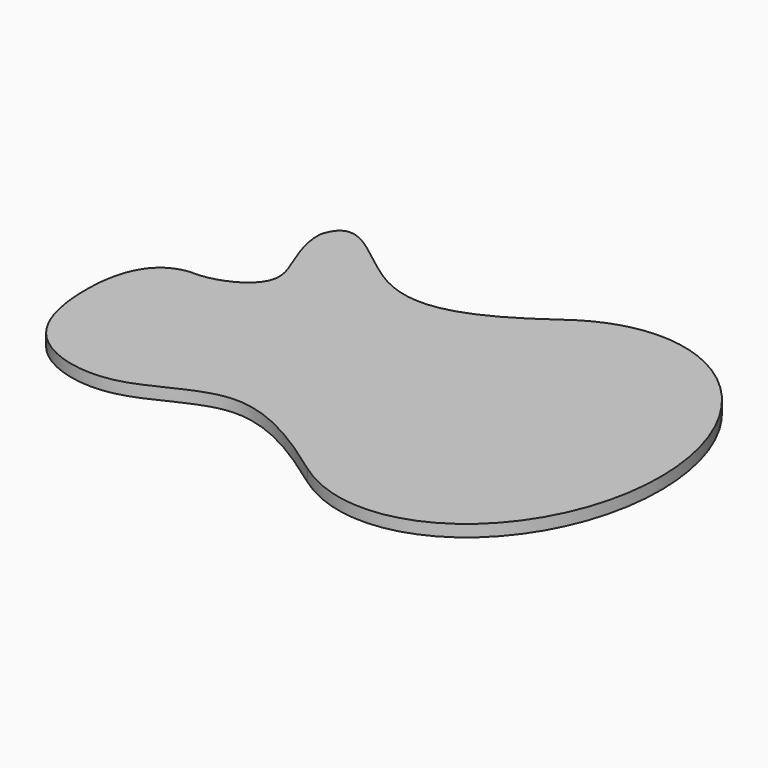
from build123d import *

# Parameters (mm, degrees)
F1_DEPTH = 8


with BuildPart() as f1:
    # F0 (on Top) → F1 (new body)
    with BuildSketch(Plane.XY):
        with BuildLine():
            add(Edge.make_bspline(
                [(71.8108263604, -123.8465007597), (47.7003894889, -106.5138372126), (-7.1023466925, -67.7010548051), (-65.7469849132, -118.3312863438), (-132.354363187, -102.6557773389), (-144.8947489305, -66.4196911039), (-145.8762223824, -43.2833050614)],
                knots=[0, 0, 0, 0, 0.2870393338, 0.537090623, 0.7679648384, 1, 1, 1, 1], degree=3))
            add(Edge.make_bspline(
                [(71.8108263604, -123.8465007597), (221.9776217834, -231.7995748847), (221.9776217834, -15.5333050614), (221.9776217834, 200.732964762), (71.8108263604, 92.7798906369)],
                knots=[2.6189550017, 2.6189550017, 2.6189550017, 4.7123889804, 4.7123889804, 6.805822959, 6.805822959, 6.805822959], degree=2, weights=[1, 0.500416121, 1, 0.500416121, 1]))
            add(Edge.make_bspline(
                [(71.8108263604, 92.7798906369), (32.8723456502, 64.787494425), (-21.3027110814, 39.7461116108), (-81.2909620858, 117.5857035406), (-89.3733802445, 87.9502004857)],
                knots=[0, 0, 0, 0, 0.5650436037, 1, 1, 1, 1], degree=3))
            add(Edge.make_bspline(
                [(-89.3733802445, 87.9502004857), (-90.0934642677, 65.0933156509), (-57.859468156, 30.7219399995), (-99.6368888097, 11.3485391097), (-115.4622438558, 12.2166949386)],
                knots=[0, 0, 0, 0, 0.5319080677, 1, 1, 1, 1], degree=3))
            add(Edge.make_bspline(
                [(-115.4622438558, 12.2166949386), (-140.0598439582, 10.2222937221), (-147.0534109131, -15.5333050614), (-145.8762223824, -43.2833050614)],
                knots=[0, 0, 0, 0, 63.2871242025, 63.2871242025, 63.2871242025, 63.2871242025], degree=3))
        make_face()
        with BuildLine():
            add(Edge.make_bspline(
                [(-81.4262804577, 86.6857544237), (-81.4396250825, 86.2899525598), (-81.470808458, 84.4412359429), (-81.2371444329, 80.3732443352), (-79.8996394846, 74.5622458053), (-77.7739796116, 68.1004270996), (-75.1889101521, 61.6875748493), (-72.6363769897, 55.6379909817), (-70.5528201855, 50.214885946), (-69.2861786808, 45.7296293686), (-68.4936431345, 42.0817923462), (-68.1698884875, 39.0929607397), (-68.1533657536, 36.6406286998), (-68.2570236145, 34.6616403838), (-68.4737574041, 33.0838263382), (-68.7291671623, 31.8176398216), (-68.9833432916, 30.7603115144), (-69.2894446793, 29.7143907955), (-69.7010474162, 28.4802252803), (-70.3057430461, 26.9847588782), (-71.2217272744, 25.180071771), (-72.5057098447, 22.996441344), (-74.3801649871, 20.4643430051), (-77.1315209855, 17.5971889856), (-80.926011463, 14.2754710831), (-86.2805957531, 10.7907129486), (-92.9455256658, 7.7447804381), (-100.4062506896, 5.4313702506), (-107.2615908321, 4.1555616419), (-112.3230611682, 4.0215517798), (-114.7617028131, 4.1430335828), (-115.474366372, 4.1953856873)],
                knots=[1.0136586156, 1.0136586156, 1.0136586156, 1.0136586156, 2.2016566853, 6.5591151943, 13.1979354067, 20.0157728224, 26.9584341349, 33.9306395999, 39.7192874549, 44.3702545919, 47.8991910145, 50.9066466506, 53.369227998, 55.2496065506, 56.847005284, 58.1419089398, 59.1235009163, 60.1084144557, 61.4103265818, 63.0253022922, 64.9424016715, 67.4766146145, 70.6177002822, 74.3676557464, 79.3769786716, 85.7174213089, 93.458168517, 101.2822181349, 109.1089736004, 114.2877981192, 116.4315649936, 116.4315649936, 116.4315649936, 116.4315649936], degree=3))
            add(Edge.make_bspline(
                [(72.8103885596, 83.6341241639), (71.1240314332, 82.4184487748), (65.3211296449, 78.2511465746), (54.3822197437, 70.6703789871), (40.5843185437, 63.3369671226), (27.1044447549, 57.4124251533), (15.6068408566, 53.964757392), (5.3548644478, 52.6151050201), (-2.8177310259, 52.7103819348), (-9.6197612713, 53.363557714), (-15.7305931996, 54.5996218363), (-21.4732164128, 56.31783797), (-26.4693776174, 58.366991406), (-30.2671336771, 60.2223905595), (-33.0718752326, 61.7320886712), (-35.2053892899, 62.9792168629), (-37.3369452365, 64.2673631998), (-39.7615979324, 65.8275673276), (-42.7778265582, 67.9000785118), (-46.5332653234, 70.5849117526), (-51.0723794993, 74.0383260586), (-56.0224963865, 77.9290754702), (-61.0223620617, 81.8442891195), (-65.7064727807, 85.3502794992), (-69.7594173643, 88.139955985), (-72.9865417062, 89.9814861225), (-75.2118467434, 90.9665662194), (-76.6921868128, 91.4830508838), (-77.6909621365, 91.7169743843), (-78.3366022017, 91.7578979554), (-78.6767300882, 91.7470455298), (-78.7973913091, 91.6896137336), (-78.92482237, 91.6464959623), (-79.1937851984, 91.3963059685), (-79.6818827943, 90.8264140362), (-80.3159105632, 89.7215409417), (-80.9369473577, 88.2993059967), (-81.2772034526, 87.2085598356), (-81.4244737614, 86.692097536), (-81.4262804577, 86.6857544237)],
                knots=[4.5292135135, 4.5292135135, 4.5292135135, 4.5292135135, 10.7658667308, 25.9500108525, 44.4238690912, 57.5330245622, 70.0845168555, 80.2898579631, 88.4222588801, 94.5557392843, 100.7652771107, 107.0947805516, 112.5088206902, 116.9457400715, 119.7701488038, 122.0625237383, 124.3588459686, 127.2414612751, 130.7107153436, 135.3368293125, 141.0894801607, 147.8190536406, 154.2256313175, 160.1398760262, 165.3706560057, 168.9759235223, 171.2693919986, 172.6578901032, 173.6814113013, 174.3231622883, 174.6136969662, 174.6729508701, 174.7225491593, 175.0159838788, 175.7405361192, 176.9913533667, 178.804034025, 180.3944536329, 180.4142282457, 180.4142282457, 180.4142282457, 180.4142282457], degree=3))
            add(Edge.make_bspline(
                [(72.8103885596, 83.6341241639), (72.7317618823, 83.5699644288), (70.9554937476, 82.1155753179), (67.9804833382, 79.4874285922), (64.1756082657, 75.8169878196), (61.2913248025, 72.7059934358), (59.0477069928, 70.0999739159), (57.2057633336, 67.8641883266), (55.4110672881, 65.56108087), (53.3041635287, 62.7354150513), (50.7805389552, 59.0881516023), (47.799656336, 54.2715974255), (44.2346711733, 47.9787195772), (40.2649118491, 39.7160179142), (36.5713092348, 29.8478370438), (33.5979528322, 19.5919068023), (31.7307948184, 10.2422116085), (30.6840668384, 2.616404127), (30.0568619889, -3.4886245577), (29.7723767309, -8.3519176651), (29.6597520537, -12.2635801323), (29.6233030189, -15.5333050614), (29.6597520537, -18.8030299904), (29.7723767309, -22.7146924576), (30.0568619889, -27.577985565), (30.6840668384, -33.6830142497), (31.7307948184, -41.3088217312), (33.5979528322, -50.658516925), (36.5713092348, -60.9144471666), (40.2649118491, -70.7826280369), (44.2346711733, -79.0453296999), (47.799656336, -85.3382075482), (50.7805389552, -90.154761725), (53.3041635287, -93.802025174), (55.4110672881, -96.6276909927), (57.2057633336, -98.9307984493), (59.0477069928, -101.1665840385), (61.2913248025, -103.7726035588), (64.1756082657, -106.8835979408), (67.9804833382, -110.5540387225), (71.0158561736, -113.2355100421), (72.8564442573, -114.7385263129), (72.9977731483, -114.8532271387)],
                knots=[55.4205486123, 55.4205486123, 55.4205486123, 55.4205486123, 55.7249011544, 62.305727762, 67.3238088056, 71.5787205888, 75.0272954709, 77.639141403, 80.2683237903, 83.7858930003, 88.2122067644, 93.5690542346, 100.7734603115, 109.9018351329, 121.0375002369, 132.3448319226, 141.8998601689, 149.6118137579, 155.4302714584, 160.3068693677, 164.2227012809, 167.1693695094, 170.1160377378, 174.0318696511, 178.9084675603, 184.7269252608, 192.4388788498, 201.9939070962, 213.3012387819, 224.4369038858, 233.5652787073, 240.7696847841, 246.1265322543, 250.5528460185, 254.0704152284, 256.6995976157, 259.3114435479, 262.76001843, 267.0149302132, 272.0330112567, 278.6138378644, 279.1597054143, 279.1597054143, 279.1597054143, 279.1597054143], degree=3))
            add(Edge.make_bspline(
                [(72.9977731483, -114.8532271387), (72.4056865049, -114.4263580428), (69.0464376439, -111.9992044047), (61.9105909681, -106.8036530478), (52.1940425374, -100.414675291), (42.2398177459, -94.2326232769), (33.0541391905, -89.1692992659), (24.2243642947, -84.9672989241), (16.2683766941, -82.0032951161), (9.8318873834, -80.2250290854), (4.463169856, -79.0636225581), (-0.1263073791, -78.4111921814), (-4.1937519975, -78.1649162686), (-7.7060356334, -78.20526396), (-11.1805991563, -78.3727848605), (-15.105690951, -78.8390498977), (-19.429069468, -79.71105596), (-23.8718019577, -80.9066029792), (-28.6468717479, -82.5067792162), (-34.2116599911, -84.6249302975), (-40.8658871469, -87.6398905134), (-47.690965404, -91.0045722285), (-53.9322172369, -94.031755035), (-58.8517886529, -96.1862154004), (-62.8636912858, -97.8099974599), (-66.2287548358, -99.0112055596), (-69.174479199, -99.8882996602), (-71.7101157046, -100.5041409348), (-74.2391141536, -101.045908585), (-77.1889902033, -101.5211815466), (-80.5636006609, -101.8380782168), (-84.1498166568, -101.9648655282), (-88.1283425241, -101.8479910003), (-92.8713789939, -101.4573804411), (-98.6786686768, -100.4434986326), (-104.6143126843, -98.6675537845), (-109.8122869472, -96.3889800651), (-113.6612373405, -94.2262164294), (-116.6721363111, -92.2928397642), (-119.445929644, -90.1897015323), (-122.5417365002, -87.5069010735), (-126.0053703089, -83.7372187502), (-129.3000799141, -78.8269050802), (-132.2206720517, -72.9997696435), (-134.760402105, -65.6917432119), (-136.8528161109, -57.6024378465), (-137.649866694, -49.6245863229), (-137.8414579174, -44.9060106494), (-137.8834109174, -42.9442403412)],
                knots=[4.2858061399, 4.2858061399, 4.2858061399, 4.2858061399, 6.4754935696, 16.7181495974, 30.7634466026, 41.3498570357, 51.8646712584, 62.2141493558, 70.6575747754, 77.2977144197, 82.2304258348, 87.1280777725, 91.1888826436, 94.4417008039, 97.6615312024, 101.6210664508, 106.2864985952, 110.880412158, 115.4145221345, 121.3894131446, 128.7352744437, 137.3194350468, 144.219174491, 149.5422059689, 153.4280250406, 157.2015215054, 160.2566826573, 162.6437031168, 165.0279610064, 168.0144585226, 171.6015387383, 175.1893400883, 178.772742133, 183.5366693447, 189.4556710281, 196.4255332119, 202.067982696, 206.4456583082, 209.6586104968, 212.7949457303, 216.8805616296, 221.934808933, 228.1024059287, 234.5573044306, 241.4332004742, 251.2825478576, 259.5402388761, 265.4359196068, 265.4359196068, 265.4359196068, 265.4359196068], degree=3))
            add(Edge.make_bspline(
                [(-115.474366372, 4.1953856873), (-115.654699102, 4.1804409153), (-116.5836359717, 4.0950636678), (-118.5079216061, 3.8241612148), (-121.094735833, 3.0439396902), (-123.6838235375, 1.8597581111), (-125.9853889989, 0.3481336416), (-128.0619952594, -1.4951736511), (-129.9535460087, -3.6932073495), (-131.8514714309, -6.5803447016), (-133.9637161202, -10.6180046655), (-136.0486166412, -16.5975276115), (-137.4710871628, -24.3656867863), (-138.1549681717, -32.3234699475), (-138.079170547, -38.6118374717), (-137.939859331, -41.8534729549), (-137.8834109174, -42.9442403412)],
                knots=[0.6605528161, 0.6605528161, 0.6605528161, 0.6605528161, 1.2032828879, 3.4574616871, 6.4791602651, 9.2718264149, 11.9726703823, 14.7076610425, 17.5762809491, 20.6455316793, 25.0544251668, 31.2157003257, 39.5600454386, 48.6812593878, 55.1351477368, 58.4131045259, 58.4131045259, 58.4131045259, 58.4131045259], degree=3))
        make_face(mode=Mode.SUBTRACT)
        with BuildLine():
            add(Edge.make_bspline(
                [(72.8103885596, 83.6341241639), (71.1240314332, 82.4184487748), (65.3211296449, 78.2511465746), (54.3822197437, 70.6703789871), (40.5843185437, 63.3369671226), (27.1044447549, 57.4124251533), (15.6068408566, 53.964757392), (5.3548644478, 52.6151050201), (-2.8177310259, 52.7103819348), (-9.6197612713, 53.363557714), (-15.7305931996, 54.5996218363), (-21.4732164128, 56.31783797), (-26.4693776174, 58.366991406), (-30.2671336771, 60.2223905595), (-33.0718752326, 61.7320886712), (-35.2053892899, 62.9792168629), (-37.3369452365, 64.2673631998), (-39.7615979324, 65.8275673276), (-42.7778265582, 67.9000785118), (-46.5332653234, 70.5849117526), (-51.0723794993, 74.0383260586), (-56.0224963865, 77.9290754702), (-61.0223620617, 81.8442891195), (-65.7064727807, 85.3502794992), (-69.7594173643, 88.139955985), (-72.9865417062, 89.9814861225), (-75.2118467434, 90.9665662194), (-76.6921868128, 91.4830508838), (-77.6909621365, 91.7169743843), (-78.3366022017, 91.7578979554), (-78.6767300882, 91.7470455298), (-78.7973913091, 91.6896137336), (-78.92482237, 91.6464959623), (-79.1937851984, 91.3963059685), (-79.6818827943, 90.8264140362), (-80.3159105632, 89.7215409417), (-80.9369473577, 88.2993059967), (-81.2772034526, 87.2085598356), (-81.4244737614, 86.692097536), (-81.4262804577, 86.6857544237)],
                knots=[4.5292135135, 4.5292135135, 4.5292135135, 4.5292135135, 10.7658667308, 25.9500108525, 44.4238690912, 57.5330245622, 70.0845168555, 80.2898579631, 88.4222588801, 94.5557392843, 100.7652771107, 107.0947805516, 112.5088206902, 116.9457400715, 119.7701488038, 122.0625237383, 124.3588459686, 127.2414612751, 130.7107153436, 135.3368293125, 141.0894801607, 147.8190536406, 154.2256313175, 160.1398760262, 165.3706560057, 168.9759235223, 171.2693919986, 172.6578901032, 173.6814113013, 174.3231622883, 174.6136969662, 174.6729508701, 174.7225491593, 175.0159838788, 175.7405361192, 176.9913533667, 178.804034025, 180.3944536329, 180.4142282457, 180.4142282457, 180.4142282457, 180.4142282457], degree=3))
            add(Edge.make_bspline(
                [(-81.4262804577, 86.6857544237), (-81.4396250825, 86.2899525598), (-81.470808458, 84.4412359429), (-81.2371444329, 80.3732443352), (-79.8996394846, 74.5622458053), (-77.7739796116, 68.1004270996), (-75.1889101521, 61.6875748493), (-72.6363769897, 55.6379909817), (-70.5528201855, 50.214885946), (-69.2861786808, 45.7296293686), (-68.4936431345, 42.0817923462), (-68.1698884875, 39.0929607397), (-68.1533657536, 36.6406286998), (-68.2570236145, 34.6616403838), (-68.4737574041, 33.0838263382), (-68.7291671623, 31.8176398216), (-68.9833432916, 30.7603115144), (-69.2894446793, 29.7143907955), (-69.7010474162, 28.4802252803), (-70.3057430461, 26.9847588782), (-71.2217272744, 25.180071771), (-72.5057098447, 22.996441344), (-74.3801649871, 20.4643430051), (-77.1315209855, 17.5971889856), (-80.926011463, 14.2754710831), (-86.2805957531, 10.7907129486), (-92.9455256658, 7.7447804381), (-100.4062506896, 5.4313702506), (-107.2615908321, 4.1555616419), (-112.3230611682, 4.0215517798), (-114.7617028131, 4.1430335828), (-115.474366372, 4.1953856873)],
                knots=[1.0136586156, 1.0136586156, 1.0136586156, 1.0136586156, 2.2016566853, 6.5591151943, 13.1979354067, 20.0157728224, 26.9584341349, 33.9306395999, 39.7192874549, 44.3702545919, 47.8991910145, 50.9066466506, 53.369227998, 55.2496065506, 56.847005284, 58.1419089398, 59.1235009163, 60.1084144557, 61.4103265818, 63.0253022922, 64.9424016715, 67.4766146145, 70.6177002822, 74.3676557464, 79.3769786716, 85.7174213089, 93.458168517, 101.2822181349, 109.1089736004, 114.2877981192, 116.4315649936, 116.4315649936, 116.4315649936, 116.4315649936], degree=3))
            add(Edge.make_bspline(
                [(-115.474366372, 4.1953856873), (-115.654699102, 4.1804409153), (-116.5836359717, 4.0950636678), (-118.5079216061, 3.8241612148), (-121.094735833, 3.0439396902), (-123.6838235375, 1.8597581111), (-125.9853889989, 0.3481336416), (-128.0619952594, -1.4951736511), (-129.9535460087, -3.6932073495), (-131.8514714309, -6.5803447016), (-133.9637161202, -10.6180046655), (-136.0486166412, -16.5975276115), (-137.4710871628, -24.3656867863), (-138.1549681717, -32.3234699475), (-138.079170547, -38.6118374717), (-137.939859331, -41.8534729549), (-137.8834109174, -42.9442403412)],
                knots=[0.6605528161, 0.6605528161, 0.6605528161, 0.6605528161, 1.2032828879, 3.4574616871, 6.4791602651, 9.2718264149, 11.9726703823, 14.7076610425, 17.5762809491, 20.6455316793, 25.0544251668, 31.2157003257, 39.5600454386, 48.6812593878, 55.1351477368, 58.4131045259, 58.4131045259, 58.4131045259, 58.4131045259], degree=3))
            add(Edge.make_bspline(
                [(72.9977731483, -114.8532271387), (72.4056865049, -114.4263580428), (69.0464376439, -111.9992044047), (61.9105909681, -106.8036530478), (52.1940425374, -100.414675291), (42.2398177459, -94.2326232769), (33.0541391905, -89.1692992659), (24.2243642947, -84.9672989241), (16.2683766941, -82.0032951161), (9.8318873834, -80.2250290854), (4.463169856, -79.0636225581), (-0.1263073791, -78.4111921814), (-4.1937519975, -78.1649162686), (-7.7060356334, -78.20526396), (-11.1805991563, -78.3727848605), (-15.105690951, -78.8390498977), (-19.429069468, -79.71105596), (-23.8718019577, -80.9066029792), (-28.6468717479, -82.5067792162), (-34.2116599911, -84.6249302975), (-40.8658871469, -87.6398905134), (-47.690965404, -91.0045722285), (-53.9322172369, -94.031755035), (-58.8517886529, -96.1862154004), (-62.8636912858, -97.8099974599), (-66.2287548358, -99.0112055596), (-69.174479199, -99.8882996602), (-71.7101157046, -100.5041409348), (-74.2391141536, -101.045908585), (-77.1889902033, -101.5211815466), (-80.5636006609, -101.8380782168), (-84.1498166568, -101.9648655282), (-88.1283425241, -101.8479910003), (-92.8713789939, -101.4573804411), (-98.6786686768, -100.4434986326), (-104.6143126843, -98.6675537845), (-109.8122869472, -96.3889800651), (-113.6612373405, -94.2262164294), (-116.6721363111, -92.2928397642), (-119.445929644, -90.1897015323), (-122.5417365002, -87.5069010735), (-126.0053703089, -83.7372187502), (-129.3000799141, -78.8269050802), (-132.2206720517, -72.9997696435), (-134.760402105, -65.6917432119), (-136.8528161109, -57.6024378465), (-137.649866694, -49.6245863229), (-137.8414579174, -44.9060106494), (-137.8834109174, -42.9442403412)],
                knots=[4.2858061399, 4.2858061399, 4.2858061399, 4.2858061399, 6.4754935696, 16.7181495974, 30.7634466026, 41.3498570357, 51.8646712584, 62.2141493558, 70.6575747754, 77.2977144197, 82.2304258348, 87.1280777725, 91.1888826436, 94.4417008039, 97.6615312024, 101.6210664508, 106.2864985952, 110.880412158, 115.4145221345, 121.3894131446, 128.7352744437, 137.3194350468, 144.219174491, 149.5422059689, 153.4280250406, 157.2015215054, 160.2566826573, 162.6437031168, 165.0279610064, 168.0144585226, 171.6015387383, 175.1893400883, 178.772742133, 183.5366693447, 189.4556710281, 196.4255332119, 202.067982696, 206.4456583082, 209.6586104968, 212.7949457303, 216.8805616296, 221.934808933, 228.1024059287, 234.5573044306, 241.4332004742, 251.2825478576, 259.5402388761, 265.4359196068, 265.4359196068, 265.4359196068, 265.4359196068], degree=3))
            add(Edge.make_bspline(
                [(72.8103885596, 83.6341241639), (72.7317618823, 83.5699644288), (70.9554937476, 82.1155753179), (67.9804833382, 79.4874285922), (64.1756082657, 75.8169878196), (61.2913248025, 72.7059934358), (59.0477069928, 70.0999739159), (57.2057633336, 67.8641883266), (55.4110672881, 65.56108087), (53.3041635287, 62.7354150513), (50.7805389552, 59.0881516023), (47.799656336, 54.2715974255), (44.2346711733, 47.9787195772), (40.2649118491, 39.7160179142), (36.5713092348, 29.8478370438), (33.5979528322, 19.5919068023), (31.7307948184, 10.2422116085), (30.6840668384, 2.616404127), (30.0568619889, -3.4886245577), (29.7723767309, -8.3519176651), (29.6597520537, -12.2635801323), (29.6233030189, -15.5333050614), (29.6597520537, -18.8030299904), (29.7723767309, -22.7146924576), (30.0568619889, -27.577985565), (30.6840668384, -33.6830142497), (31.7307948184, -41.3088217312), (33.5979528322, -50.658516925), (36.5713092348, -60.9144471666), (40.2649118491, -70.7826280369), (44.2346711733, -79.0453296999), (47.799656336, -85.3382075482), (50.7805389552, -90.154761725), (53.3041635287, -93.802025174), (55.4110672881, -96.6276909927), (57.2057633336, -98.9307984493), (59.0477069928, -101.1665840385), (61.2913248025, -103.7726035588), (64.1756082657, -106.8835979408), (67.9804833382, -110.5540387225), (71.0158561736, -113.2355100421), (72.8564442573, -114.7385263129), (72.9977731483, -114.8532271387)],
                knots=[55.4205486123, 55.4205486123, 55.4205486123, 55.4205486123, 55.7249011544, 62.305727762, 67.3238088056, 71.5787205888, 75.0272954709, 77.639141403, 80.2683237903, 83.7858930003, 88.2122067644, 93.5690542346, 100.7734603115, 109.9018351329, 121.0375002369, 132.3448319226, 141.8998601689, 149.6118137579, 155.4302714584, 160.3068693677, 164.2227012809, 167.1693695094, 170.1160377378, 174.0318696511, 178.9084675603, 184.7269252608, 192.4388788498, 201.9939070962, 213.3012387819, 224.4369038858, 233.5652787073, 240.7696847841, 246.1265322543, 250.5528460185, 254.0704152284, 256.6995976157, 259.3114435479, 262.76001843, 267.0149302132, 272.0330112567, 278.6138378644, 279.1597054143, 279.1597054143, 279.1597054143, 279.1597054143], degree=3))
        make_face()
    extrude(amount=F1_DEPTH)


solid = f1.part
